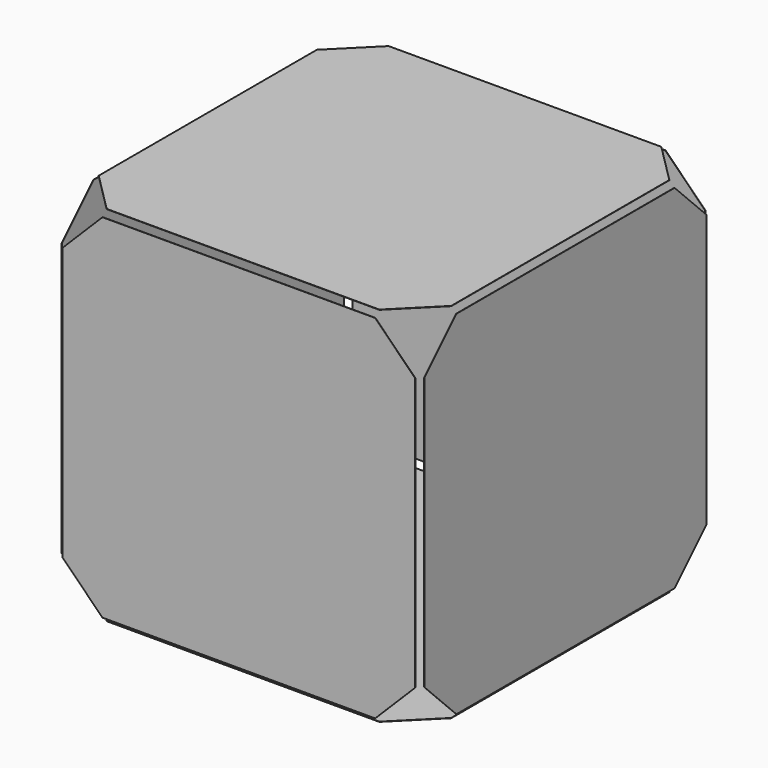
from build123d import *

# Parameters (mm, degrees)
F6_DEPTH         = 0.254
F6_COPIES2_COUNT = 2
F6_COPIES2_ANGLE = 270
F6_COPIES3_COUNT = 2
F6_COPIES3_ANGLE = 90


# Not quite as in the source:
# - a feature of the source that left no trace in its solid (it failed there, or was rolled back) is left out
# - a pattern or mirror of a feature is missing from the dataset's text; its kind, count and spacing are read off the source's solid
# - a feature names something its author has since deleted; it is built from what else it names


with BuildPart() as f6:
    # F2 (on offset) → F6 (new body)
    with BuildSketch(Plane.XZ.offset(-4.7625)):
        Polygon((9.525, 307.975), (9.525, 47.625), (47.625, 9.525), (307.975, 9.525), (346.075, 47.625), (346.075, 307.975), (307.975, 346.075), (47.625, 346.075), align=None)
    extrude(amount=F6_DEPTH)


with BuildPart() as f6_copies_1:
    # F6_copies: instance of F6
    add(f6.part.mirror(Plane(origin=(0, 0, 0), x_dir=(0, -0.7071067812, -0.7071067812), z_dir=(0, 0.7071067812, -0.7071067812))))


with BuildPart() as f6_copies1_1:
    # F6_copies1: instance of F6
    add(f6.part.mirror(Plane(origin=(0, 0, 0), x_dir=(-0.7071067812, -0.7071067812, 0), z_dir=(-0.7071067812, 0.7071067812, 0))))


with BuildPart() as f6_copies2_1:
    # F6_copies2: instance of F6
    add(f6.part.rotate(Axis((350.9645, 4.6355, 0), (0, 0, 1)), 1 * F6_COPIES2_ANGLE / (F6_COPIES2_COUNT - 1)))


with BuildPart() as f6_copies3_1:
    # F6_copies3: instance of F6
    add(f6.part.rotate(Axis((0, 4.6355, 350.9645), (1, 0, 0)), 1 * F6_COPIES3_ANGLE / (F6_COPIES3_COUNT - 1)))


with BuildPart() as f9_1:
    # F9: instance of F6
    add(f6.part.mirror(Plane.XZ.offset(-177.8)))


solid = Compound([f6.part, f6_copies_1.part, f6_copies1_1.part, f6_copies2_1.part, f6_copies3_1.part, f9_1.part])
